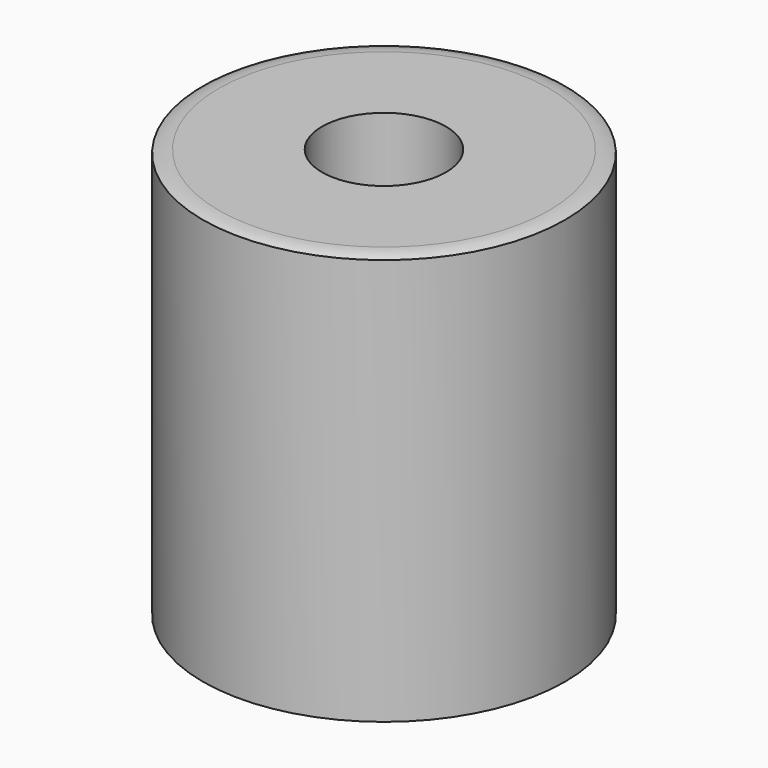
from build123d import *

# Parameters (mm, degrees)
F0_R      = 40
F0_R_2    = 35
F1_DEPTH  = 5
F2_R      = 4.99999
F3_DEPTH  = 2.5
F4_R      = 5
F5_DEPTH  = 5
F6_R      = 1.5
F7_DEPTH  = 5
F9_DEPTH  = 2.5
F10_R     = 1
F11_R     = 44.5515786246
F11_R_2   = 4.3855137127
F12_DEPTH = 6


# Not quite as in the source:
# - a fillet or chamfer is up to 0.001 mm smaller than in the source, because OpenCascade refuses the exact size


with BuildPart() as f1:
    # F0 (on Top) → F1 (new body, symmetric)
    with BuildSketch(Plane.XY):
        Circle(F0_R)
        Circle(F0_R_2, mode=Mode.SUBTRACT)
    extrude(amount=F1_DEPTH, both=True)

    # F2 (radius 5 in the source; OpenCascade refuses exactly that, so slightly less here)
    f2_edges = [f1.edges().sort_by_distance(p)[0] for p in [
        (-40, 0, 5),
        (-40, 0, -5),
    ]]
    fillet(f2_edges, radius=F2_R)

    # F0 (on Top) → F3 (join, symmetric)
    with BuildSketch(Plane.XY):
        Circle(F0_R_2)
    extrude(amount=F3_DEPTH, both=True)

    # F4 (on Top) → F5 (join, symmetric)
    with BuildSketch(Plane.XY):
        Circle(F4_R)
    extrude(amount=F5_DEPTH, both=True)

    # F6 (on Top) → F7 (cut, symmetric)
    with BuildSketch(Plane.XY):
        Circle(F6_R)
    extrude(amount=F7_DEPTH, both=True, mode=Mode.SUBTRACT)

    # F8 (on Top) → F9 (cut, symmetric)
    with BuildSketch(Plane.XY):
        with BuildLine():
            ThreePointArc((-30.0140328654, 11.8585631023), (-31.0869388877, 8.7208064041), (-31.7860568579, 5.4792206049))
            ThreePointArc((-31.7860568579, 5.4792206049), (-31.3779575205, 3.9314640765), (-29.9653471981, 3.1787174941))
            Line((-29.9653471981, 3.1787174941), (-8.8751398211, 1.5323311534))
            ThreePointArc((-8.8751398211, 1.5323311534), (-7.8337940647, 2.2616563361), (-8.3497989023, 3.4235751))
            Line((-8.3497989023, 3.4235751), (-27.2676686416, 12.89044574))
            ThreePointArc((-27.2676686416, 12.89044574), (-28.866135701, 12.9741021828), (-30.0140328654, 11.8585631023))
        make_face()
        with BuildLine():
            ThreePointArc((-30.3900590314, -11.1791820248), (-29.2627563738, -12.3155288285), (-27.6630266578, -12.2611213303))
            Line((-27.6630266578, -12.2611213303), (-8.5751781278, -3.1418300373))
            ThreePointArc((-8.5751781278, -3.1418300373), (-8.03800884, -1.9895430233), (-9.0658415198, -1.2412942754))
            Line((-9.0658415198, -1.2412942754), (-30.1826326195, -2.5016786765))
            ThreePointArc((-30.1826326195, -2.5016786765), (-31.6087739214, -3.2284636015), (-32.0451124866, -4.7684973663))
            ThreePointArc((-32.0451124866, -4.7684973663), (-31.4053980086, -8.022327389), (-30.3900590314, -11.1791820248))
        make_face()
        with BuildLine():
            ThreePointArc((-20.8518881352, -24.9077829753), (-19.3074419941, -25.328236846), (-17.9492391699, -24.4812537124))
            Line((-17.9492391699, -24.4812537124), (-5.978323086, -7.0397915232))
            ThreePointArc((-5.978323086, -7.0397915232), (-6.0892643436, -5.7732970527), (-7.3535179291, -5.6392109685))
            Line((-7.3535179291, -5.6392109685), (-25.0110032673, -17.2891314283))
            ThreePointArc((-25.0110032673, -17.2891314283), (-25.8826854016, -18.6316162874), (-25.4905488012, -20.183493933))
            ThreePointArc((-25.4905488012, -20.183493933), (-23.3096248008, -22.6815361533), (-20.8518881352, -24.9077829753))
        make_face()
        with BuildLine():
            ThreePointArc((-5.7272893582, -32.0280147088), (-4.1795328299, -31.6199153714), (-3.4267862475, -30.207305049))
            Line((-3.4267862475, -30.207305049), (-1.7803999068, -9.117097672))
            ThreePointArc((-1.7803999068, -9.117097672), (-2.5097250895, -8.0757519156), (-3.6716438534, -8.5917567532))
            Line((-3.6716438534, -8.5917567532), (-13.1385144934, -27.5096264925))
            ThreePointArc((-13.1385144934, -27.5096264925), (-13.2221709361, -29.1080935518), (-12.1066318557, -30.2559907163))
            ThreePointArc((-12.1066318557, -30.2559907163), (-8.9688751575, -31.3288967386), (-5.7272893582, -32.0280147088))
        make_face()
        with BuildLine():
            ThreePointArc((10.9311132714, -30.6320168823), (12.0674600751, -29.5047142247), (12.0130525769, -27.9049845086))
            Line((12.0130525769, -27.9049845086), (2.8937612839, -8.8171359787))
            ThreePointArc((2.8937612839, -8.8171359787), (1.7414742699, -8.2799666909), (0.993225522, -9.3077993707))
            Line((0.993225522, -9.3077993707), (2.2536099231, -30.4245904704))
            ThreePointArc((2.2536099231, -30.4245904704), (2.9803948481, -31.8507317723), (4.5204286129, -32.2870703374))
            ThreePointArc((4.5204286129, -32.2870703374), (7.7742586356, -31.6473558595), (10.9311132714, -30.6320168823))
        make_face()
        with BuildLine():
            ThreePointArc((24.6597142219, -21.0938459861), (25.0801680926, -19.549399845), (24.233184959, -18.1911970208))
            Line((24.233184959, -18.1911970208), (6.7917227698, -6.2202809368))
            ThreePointArc((6.7917227698, -6.2202809368), (5.5252282993, -6.3312221945), (5.3911422152, -7.5954757799))
            Line((5.3911422152, -7.5954757799), (17.0410626749, -25.2529611182))
            ThreePointArc((17.0410626749, -25.2529611182), (18.383547534, -26.1246432525), (19.9354251796, -25.7325066521))
            ThreePointArc((19.9354251796, -25.7325066521), (22.4334673999, -23.5515826517), (24.6597142219, -21.0938459861))
        make_face()
        with BuildLine():
            ThreePointArc((31.7799459554, -5.9692472091), (31.371846618, -4.4214906808), (29.9592362956, -3.6687440984))
            Line((29.9592362956, -3.6687440984), (8.8690289186, -2.0223577577))
            ThreePointArc((8.8690289186, -2.0223577577), (7.8276831622, -2.7516829403), (8.3436879998, -3.9136017043))
            Line((8.3436879998, -3.9136017043), (27.2615577391, -13.3804723443))
            ThreePointArc((27.2615577391, -13.3804723443), (28.8600247985, -13.464128787), (30.0079219629, -12.3485897066))
            ThreePointArc((30.0079219629, -12.3485897066), (31.0808279852, -9.2108330083), (31.7799459554, -5.9692472091))
        make_face()
        with BuildLine():
            ThreePointArc((30.3839481289, 10.6891554205), (29.2566454713, 11.8255022243), (27.6569157553, 11.7710947261))
            Line((27.6569157553, 11.7710947261), (8.5690672253, 2.651803433))
            ThreePointArc((8.5690672253, 2.651803433), (8.0318979375, 1.499516419), (9.0597306173, 0.7512676711))
            Line((9.0597306173, 0.7512676711), (30.176521717, 2.0116520722))
            ThreePointArc((30.176521717, 2.0116520722), (31.6026630189, 2.7384369973), (32.0390015841, 4.2784707621))
            ThreePointArc((32.0390015841, 4.2784707621), (31.3992871061, 7.5323007848), (30.3839481289, 10.6891554205))
        make_face()
        with BuildLine():
            ThreePointArc((20.8457772327, 24.417756371), (19.3013310916, 24.8382102418), (17.9431282674, 23.9912271081))
            Line((17.9431282674, 23.9912271081), (5.9722121835, 6.5497649189))
            ThreePointArc((5.9722121835, 6.5497649189), (6.0831534411, 5.2832704484), (7.3474070266, 5.1491843643))
            Line((7.3474070266, 5.1491843643), (25.0048923648, 16.799104824))
            ThreePointArc((25.0048923648, 16.799104824), (25.8765744991, 18.1415896832), (25.4844378987, 19.6934673287))
            ThreePointArc((25.4844378987, 19.6934673287), (23.3035138983, 22.191509549), (20.8457772327, 24.417756371))
        make_face()
        with BuildLine():
            ThreePointArc((5.7211784557, 31.5379881045), (4.1734219274, 31.1298887671), (3.420675345, 29.7172784447))
            Line((3.420675345, 29.7172784447), (1.7742890043, 8.6270710677))
            ThreePointArc((1.7742890043, 8.6270710677), (2.503614187, 7.5857253113), (3.6655329509, 8.1017301489))
            Line((3.6655329509, 8.1017301489), (13.1324035909, 27.0195998883))
            ThreePointArc((13.1324035909, 27.0195998883), (13.2160600336, 28.6180669476), (12.1005209532, 29.7659641121))
            ThreePointArc((12.1005209532, 29.7659641121), (8.9627642549, 30.8388701343), (5.7211784557, 31.5379881045))
        make_face()
        with BuildLine():
            ThreePointArc((-10.9372241739, 30.141990278), (-12.0735709776, 29.0146876204), (-12.0191634794, 27.4149579044))
            Line((-12.0191634794, 27.4149579044), (-2.8998721864, 8.3271093745))
            ThreePointArc((-2.8998721864, 8.3271093745), (-1.7475851724, 7.7899400866), (-0.9993364245, 8.8177727664))
            Line((-0.9993364245, 8.8177727664), (-2.2597208256, 29.9345638662))
            ThreePointArc((-2.2597208256, 29.9345638662), (-2.9865057506, 31.360705168), (-4.5265395155, 31.7970437332))
            ThreePointArc((-4.5265395155, 31.7970437332), (-7.7803695381, 31.1573292552), (-10.9372241739, 30.141990278))
        make_face()
        with BuildLine():
            ThreePointArc((-24.6658251244, 20.6038193818), (-25.0862789951, 19.0593732407), (-24.2392958615, 17.7011704166))
            Line((-24.2392958615, 17.7011704166), (-6.7978336723, 5.7302543326))
            ThreePointArc((-6.7978336723, 5.7302543326), (-5.5313392018, 5.8411955902), (-5.3972531177, 7.1054491757))
            Line((-5.3972531177, 7.1054491757), (-17.0471735774, 24.7629345139))
            ThreePointArc((-17.0471735774, 24.7629345139), (-18.3896584365, 25.6346166482), (-19.9415360821, 25.2424800479))
            ThreePointArc((-19.9415360821, 25.2424800479), (-22.4395783024, 23.0615560474), (-24.6658251244, 20.6038193818))
        make_face()
    extrude(amount=F9_DEPTH, both=True, mode=Mode.SUBTRACT)

    # F10
    f10_edges = [f1.edges().sort_by_distance(p)[0] for p in [
        (-19.420244, 2.355524, 2.5),
        (-17.808734, 8.15701, 2.5),
        (-35, 0, -2.5),
        (23.303514, 22.19151, -2.5),
        (7.774259, -31.647356, -2.5),
        (15.512454, -12.205739, -2.5),
        (11.216102, -16.424218, -2.5),
        (25.080168, -19.5494, -2.5),
        (17.802623, -8.647037, -2.5),
        (-8.405079, -18.050692, -2.5),
        (-8.968875, -31.328897, -2.5),
        (7.453407, -18.36106, -2.5),
        (-25.086279, 19.059373, -2.5),
        (-12.073571, 29.014688, -2.5),
        (-23.309625, -22.681536, -2.5),
        (-16.182261, -11.464171, -2.5),
        (-31.086939, 8.720806, -2.5),
        (-11.963781, -15.760523, -2.5),
        (-29.262756, -12.315529, -2.5),
        (-31.405398, -8.022327, -2.5),
        (-18.119102, -7.701476, -2.5),
        (-22.439578, 23.061556, -2.5),
        (-17.808734, 8.15701, -2.5),
        (-11.222213, 15.934192, -2.5),
        (8.962764, 30.83887, -2.5),
        (16.17615, 10.974145, -2.5),
        (31.080828, -9.210833, -2.5),
        (18.383548, -26.124643, -2.5),
        (18.112991, 7.211449, -2.5),
        (31.399287, 7.532301, -2.5),
        (11.95767, 15.270496, -2.5),
        (2.503614, 7.585725, -2.5),
        (-7.78037, 31.157329, -2.5),
        (22.433467, -23.551583, -2.5),
        (-2.986506, 31.360705, -2.5),
        (-13.222171, -29.108094, -2.5),
        (-7.459518, 17.871034, -2.5),
        (-25.882685, -18.631616, -2.5),
        (8.398968, 17.560665, -2.5),
        (-5, 0, -5),
        (16.17615, 10.974145, 2.5),
        (25.876574, 18.14159, -2.5),
        (-2.603593, -19.662201, -2.5),
        (1.623418, -19.866195, 2.5),
        (1.623418, -19.866195, -2.5),
        (7.774259, -31.647356, 2.5),
        (11.216102, -16.424218, 2.5),
        (31.371847, -4.421491, -2.5),
        (19.618126, 1.38146, -2.5),
        (29.256645, 11.825502, -2.5),
        (-8.405079, -18.050692, 2.5),
        (-19.941536, 25.24248, 0),
        (-35, 0, 2.5),
        (-8.968875, -31.328897, 2.5),
        (-4.179533, -31.619915, -2.5),
        (7.453407, -18.36106, 2.5),
        (-11.222213, 15.934192, 2.5),
        (-15.518565, 11.715712, -2.5),
        (-5.531339, 5.841196, -2.5),
        (-28.866136, 12.974102, -2.5),
        (-15.518565, 11.715712, 2.5),
        (-25.882685, -18.631616, 2.5),
        (24.233185, -18.191197, 0),
        (4.520429, -32.28707, 0),
        (-23.309625, -22.681536, 2.5),
        (10.931113, -30.632017, 0),
        (-16.182261, -11.464171, 2.5),
        (-6.089264, -5.773297, -2.5),
        (5.721178, 31.537988, 0),
        (-12.106632, -30.255991, 0),
        (-11.963781, -15.760523, 2.5),
        (-31.608774, -3.228464, -2.5),
        (20.845777, 24.417756, 0),
        (-31.405398, -8.022327, 2.5),
        (-19.624237, -1.871486, -2.5),
        (-8.038009, -1.989543, -2.5),
        (-31.086939, 8.720806, 2.5),
        (-25.086279, 19.059373, 2.5),
        (-18.389658, 25.634617, -2.5),
        (-22.439578, 23.061556, 2.5),
        (5.391142, -7.595476, 0),
        (17.041063, -25.252961, 0),
        (-31.377958, 3.931464, -2.5),
        (24.659714, -21.093846, 0),
        (19.935425, -25.732507, 0),
        (27.261558, -13.380472, 0),
        (-5, 0, 2.5),
        (-7.459518, 17.871034, 2.5),
        (-30.014033, 11.858563, 0),
        (4.173422, 31.129889, -2.5),
        (13.21606, 28.618067, -2.5),
        (8.962764, 30.83887, 2.5),
        (2.597482, 19.172175, -2.5),
        (-4.52654, 31.797044, 0),
        (19.301331, 24.83821, -2.5),
        (-10.937224, 30.14199, 0),
        (-2.259721, 29.934564, 0),
        (-12.019163, 27.414958, 0),
        (23.303514, 22.19151, 2.5),
        (3.665533, 8.10173, 0),
        (-27.663027, -12.261121, 0),
        (-30.390059, -11.179182, 0),
        (-25.011003, -17.289131, 0),
        (-20.851888, -24.907783, 0),
        (-25.490549, -20.183494, 0),
        (-3.671644, -8.591757, 0),
        (22.433467, -23.551583, 2.5),
        (2.893761, -8.817136, 0),
        (25.080168, -19.5494, 2.5),
        (-5, 0, -2.5),
        (19.414133, -2.845551, 2.5),
        (19.414133, -2.845551, -2.5),
        (18.383548, -26.124643, 2.5),
        (-2.509725, -8.075752, -2.5),
        (18.112991, 7.211449, 2.5),
        (6.083153, 5.28327, -2.5),
        (8.398968, 17.560665, 2.5),
        (17.802623, -8.647037, 2.5),
        (15.512454, -12.205739, 2.5),
        (31.080828, -9.210833, 2.5),
        (6.791723, -6.220281, 0),
        (1.741474, -8.279967, -2.5),
        (-7.833794, 2.261656, -2.5),
        (28.860025, -13.464129, -2.5),
        (11.95767, 15.270496, 2.5),
        (-1.747585, 7.78994, -2.5),
        (-7.78037, 31.157329, 2.5),
        (-27.267669, 12.890446, 0),
        (-19.307442, -25.328237, -2.5),
        (8.343688, -3.913602, 0),
        (19.618126, 1.38146, 2.5),
        (-13.138514, -27.509626, 0),
        (31.602663, 2.738437, -2.5),
        (12.06746, -29.504714, -2.5),
        (-18.119102, -7.701476, 2.5),
        (2.980395, -31.850732, -2.5),
        (-19.624237, -1.871486, 2.5),
        (7.827683, -2.751683, -2.5),
        (5.525228, -6.331222, -2.5),
        (-7.833794, 2.261656, 2.5),
        (1.741474, -8.279967, 2.5),
        (2.980395, -31.850732, 2.5),
        (12.06746, -29.504714, 2.5),
        (-19.307442, -25.328237, 2.5),
        (-2.603593, -19.662201, 2.5),
        (-2.509725, -8.075752, 2.5),
        (-8.87514, 1.532331, 0),
        (-13.222171, -29.108094, 2.5),
        (-4.179533, -31.619915, 2.5),
        (-31.786057, 5.479221, 0),
        (-8.349799, 3.423575, 0),
        (-5.531339, 5.841196, 2.5),
        (2.25361, -30.42459, 0),
        (-6.089264, -5.773297, 2.5),
        (12.013053, -27.904985, 0),
        (-29.262756, -12.315529, 2.5),
        (25.484438, 19.693467, 0),
        (-31.608774, -3.228464, 2.5),
        (32.039002, 4.278471, 0),
        (30.383948, 10.689155, 0),
        (-8.038009, -1.989543, 2.5),
        (9.059731, 0.751268, 0),
        (-28.866136, 12.974102, 2.5),
        (-18.389658, 25.634617, 2.5),
        (31.779946, -5.969247, 0),
        (30.007922, -12.34859, 0),
        (27.656916, 11.771095, 0),
        (4.173422, 31.129889, 2.5),
        (-6.797834, 5.730254, 0),
        (2.597482, 19.172175, 2.5),
        (19.301331, 24.83821, 2.5),
        (-19.420244, 2.355524, -2.5),
        (25.876574, 18.14159, 2.5),
        (-29.965347, 3.178717, 0),
        (6.083153, 5.28327, 2.5),
        (29.959236, -3.668744, 0),
        (-5.397253, 7.105449, 0),
        (2.503614, 7.585725, 2.5),
        (-8.575178, -3.14183, 0),
        (-9.065842, -1.241294, 0),
        (-30.182633, -2.501679, 0),
        (-32.045112, -4.768497, 0),
        (-17.949239, -24.481254, 0),
        (-5.978323, -7.039792, 0),
        (-7.353518, -5.639211, 0),
        (12.100521, 29.765964, 0),
        (-3.426786, -30.207305, 0),
        (-1.7804, -9.117098, 0),
        (30.176522, 2.011652, 0),
        (31.371847, -4.421491, 2.5),
        (25.004892, 16.799105, 0),
        (13.21606, 28.618067, 2.5),
        (-24.665825, 20.603819, 0),
        (17.943128, 23.991227, 0),
        (31.399287, 7.532301, 2.5),
        (8.869029, -2.022358, 0),
        (-5.727289, -32.028015, 0),
        (28.860025, -13.464129, 2.5),
        (29.256645, 11.825502, 2.5),
        (13.132404, 27.0196, 0),
        (5.525228, -6.331222, 2.5),
        (-1.629529, 19.376168, 2.5),
        (-1.629529, 19.376168, -2.5),
        (5.972212, 6.549765, 0),
        (1.774289, 8.627071, 0),
        (8.031898, 1.499516, 2.5),
        (8.031898, 1.499516, -2.5),
        (-2.986506, 31.360705, 2.5),
        (3.420675, 29.717278, 0),
        (-5, 0, 5),
        (7.347407, 5.149184, 0),
        (-12.073571, 29.014688, 2.5),
        (-31.377958, 3.931464, 2.5),
        (7.827683, -2.751683, 2.5),
        (-17.047174, 24.762935, 0),
        (0.993226, -9.307799, 0),
        (-24.239296, 17.70117, 0),
        (31.602663, 2.738437, 2.5),
        (-0.999336, 8.817773, 0),
        (-1.747585, 7.78994, 2.5),
        (-2.899872, 8.327109, 0),
        (8.569067, 2.651803, 0),
    ]]
    fillet(f10_edges, radius=F10_R)

    # F11 (on Top) → F12 (cut, symmetric)
    with BuildSketch(Plane.XY):
        Circle(F11_R)
        Circle(F11_R_2, mode=Mode.SUBTRACT)
    extrude(amount=F12_DEPTH, both=True, mode=Mode.SUBTRACT)


solid = f1.part
